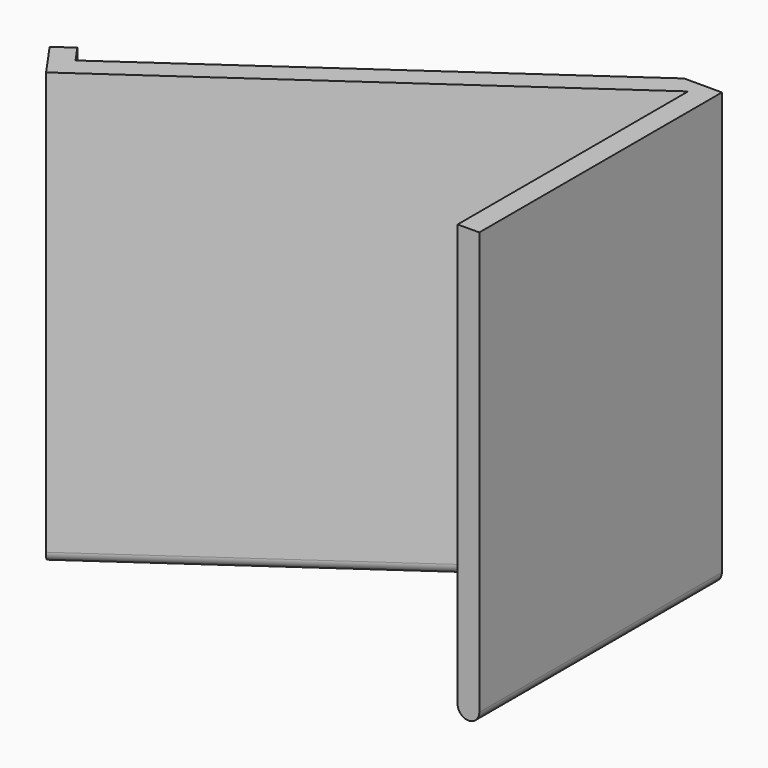
from build123d import *

# Parameters (mm, degrees)
F1_DEPTH      = 50
F1_DEPTH_BACK = 50
F2_T1_DEPTH   = 82.5
F2_T3_DEPTH   = 116.1726990145
F2_T5_DEPTH   = 11.25
F2_T10_DEPTH  = 79
F2_T15_DEPTH  = 128.4622783495
F2_T21_DEPTH  = 128.4622783495
F2_T25_DEPTH  = 79
F2_T32_DEPTH  = 122.4226990145
F2_T36_DEPTH  = 17.5


# Not quite as in the source:
# - a fillet or chamfer that OpenCascade refuses, or shapes differently, is made with other operations: its cross-section is extruded or revolved along the edge and cut away or added


with BuildPart() as f1:
    # F0 (on Top) → F1 (new body, two sides)
    with BuildSketch(Plane.XY) as f1_sk:
        Polygon((50, 35), (41.281031703, 35), (-48.7711521192, -28.0365286756), (-50, -26.281031703), (-51.638463841, -23.940369073), (-55.7346234436, -26.8076807948), (-52.8673117218, -30.9038403974), (-50, -35), (45, 31.5), (45, -35), (50, -35), align=None)
    extrude(amount=F1_DEPTH)
    extrude(f1_sk.sketch, amount=-F1_DEPTH_BACK)

    # F2: fillet of radius 2.5 on 5 edges, made by hand

    # F2_s2 → F2_t1 (cut)
    with BuildSketch(Plane.XZ.offset(-41.25)):
        with BuildLine():
            ThreePointArc((47.5, -50), (49.267766953, -49.267766953), (50, -47.5))
            Line((50, -47.5), (50, -50))
            Line((50, -50), (47.5, -50))
        make_face()
    extrude(amount=F2_T1_DEPTH, mode=Mode.SUBTRACT)

    # F2_s4 → F2_t3 (cut)
    with BuildSketch(Plane(origin=(49.2685429281, 34.4879800497, 0), x_dir=(0, 0, 1), z_dir=(-0.8192319205, -0.5734623444, 0))):
        with BuildLine():
            ThreePointArc((-50, 2.5), (-49.267766953, 4.267766953), (-47.5, 5))
            Line((-47.5, 5), (-50, 5))
            Line((-50, 5), (-50, 2.5))
        make_face()
    extrude(amount=F2_T3_DEPTH, mode=Mode.SUBTRACT)

    # F2_s6 → F2_t5 (cut)
    with BuildSketch(Plane(origin=(-2.8673117218, 4.0961596026, 0), x_dir=(0, 0, 1), z_dir=(-0.5734623444, 0.8192319205, 0))):
        with BuildLine():
            ThreePointArc((-50, -58.5327780787), (-49.267766953, -56.7650111257), (-47.5, -56.0327780787))
            Line((-47.5, -56.0327780787), (-50, -56.0327780787))
            Line((-50, -56.0327780787), (-50, -58.5327780787))
        make_face()
    extrude(amount=F2_T5_DEPTH, mode=Mode.SUBTRACT)


with BuildPart() as f2_tool8:
    # F2_s9 → F2_t10 (new body)
    with BuildSketch(Plane.XZ.offset(-37.75)):
        with BuildLine():
            ThreePointArc((47.5, -50), (45.732233047, -49.267766953), (45, -47.5))
            Line((45, -47.5), (45, -50))
            Line((45, -50), (47.5, -50))
        make_face()
    extrude(amount=F2_T10_DEPTH)

    split(bisect_by=Plane(origin=(0, 0, 0), x_dir=(0, 0, 1), z_dir=(0.5734623444, -0.8192319205, 0)), keep=Keep.TOP)


with BuildPart() as f1_1:
    add(f1.part)

    # F2_t7: cut F2_tool8
    add(f2_tool8.part, mode=Mode.SUBTRACT)


with BuildPart() as f2_tool13:
    # F2_s14 → F2_t15 (new body)
    with BuildSketch(Plane(origin=(-55.1201995032, -38.5841396523, 0), x_dir=(0, 0, 1), z_dir=(0.8192319205, 0.5734623444, 0))):
        with BuildLine():
            ThreePointArc((-47.5, 0), (-49.267766953, -0.732233047), (-50, -2.5))
            Line((-50, -2.5), (-50, 0))
            Line((-50, 0), (-47.5, 0))
        make_face()
    extrude(amount=F2_T15_DEPTH)

    split(bisect_by=Plane.YZ.offset(45), keep=Keep.BOTTOM)


with BuildPart() as f1_2:
    add(f1_1.part)

    # F2_t12: cut F2_tool13
    add(f2_tool13.part, mode=Mode.SUBTRACT)


with BuildPart() as f2_tool19:
    # F2_s20 → F2_t21 (new body)
    with BuildSketch(Plane(origin=(-55.1201995032, -38.5841396523, 0), x_dir=(0, 0, 1), z_dir=(0.8192319205, 0.5734623444, 0))):
        with BuildLine():
            ThreePointArc((-47.5, 0), (-49.267766953, -0.732233047), (-50, -2.5))
            Line((-50, -2.5), (-50, 0))
            Line((-50, 0), (-47.5, 0))
        make_face()
    extrude(amount=F2_T21_DEPTH)

    split(bisect_by=Plane.YZ.offset(45), keep=Keep.TOP)


with BuildPart() as f2_tool23:
    # F2_s24 → F2_t25 (new body)
    with BuildSketch(Plane.XZ.offset(-37.75)):
        with BuildLine():
            ThreePointArc((47.5, -50), (45.732233047, -49.267766953), (45, -47.5))
            Line((45, -47.5), (45, -50))
            Line((45, -50), (47.5, -50))
        make_face()
    extrude(amount=F2_T25_DEPTH)

    split(bisect_by=Plane(origin=(0, 0, 0), x_dir=(0, 0, 1), z_dir=(-0.5734623444, 0.8192319205, 0)), keep=Keep.TOP)


with BuildPart() as f2_tool19_1:
    add(f2_tool19.part)

    # F2_t27: intersect F2_tool23
    add(f2_tool23.part, mode=Mode.INTERSECT)


with BuildPart() as f1_3:
    add(f1_2.part)

    # F2_t17: cut F2_tool19
    add(f2_tool19_1.part, mode=Mode.SUBTRACT)


with BuildPart() as f2_tool30:
    # F2_s31 → F2_t32 (new body)
    with BuildSketch(Plane(origin=(49.2685429281, 34.4879800497, 0), x_dir=(0, 0, 1), z_dir=(-0.8192319205, -0.5734623444, 0))):
        with BuildLine():
            ThreePointArc((-50, 2.5), (-49.267766953, 4.267766953), (-47.5, 5))
            Line((-47.5, 5), (-50, 5))
            Line((-50, 5), (-50, 2.5))
        make_face()
    extrude(amount=F2_T32_DEPTH)

    split(bisect_by=Plane(origin=(-45.9038403974, -32.1326882782, 0), x_dir=(0, 0, 1), z_dir=(-0.8192319205, -0.5734623444, 0)), keep=Keep.TOP)


with BuildPart() as f2_tool34:
    # F2_s35 → F2_t36 (new body)
    with BuildSketch(Plane(origin=(0.7168279305, -1.0240399006, 0), x_dir=(0, 0, 1), z_dir=(-0.5734623444, 0.8192319205, 0))):
        with BuildLine():
            ThreePointArc((-50, -58.5327780787), (-49.267766953, -56.7650111257), (-47.5, -56.0327780787))
            Line((-47.5, -56.0327780787), (-50, -56.0327780787))
            Line((-50, -56.0327780787), (-50, -58.5327780787))
        make_face()
    extrude(amount=F2_T36_DEPTH)

    split(bisect_by=Plane(origin=(-2.8673117218, 4.0961596026, 0), x_dir=(0, 0, 1), z_dir=(0.5734623444, -0.8192319205, 0)), keep=Keep.TOP)


with BuildPart() as f2_tool30_1:
    add(f2_tool30.part)

    # F2_t38: intersect F2_tool34
    add(f2_tool34.part, mode=Mode.INTERSECT)


with BuildPart() as f1_4:
    add(f1_3.part)

    # F2_t28: cut F2_tool30
    add(f2_tool30_1.part, mode=Mode.SUBTRACT)


solid = f1_4.part
